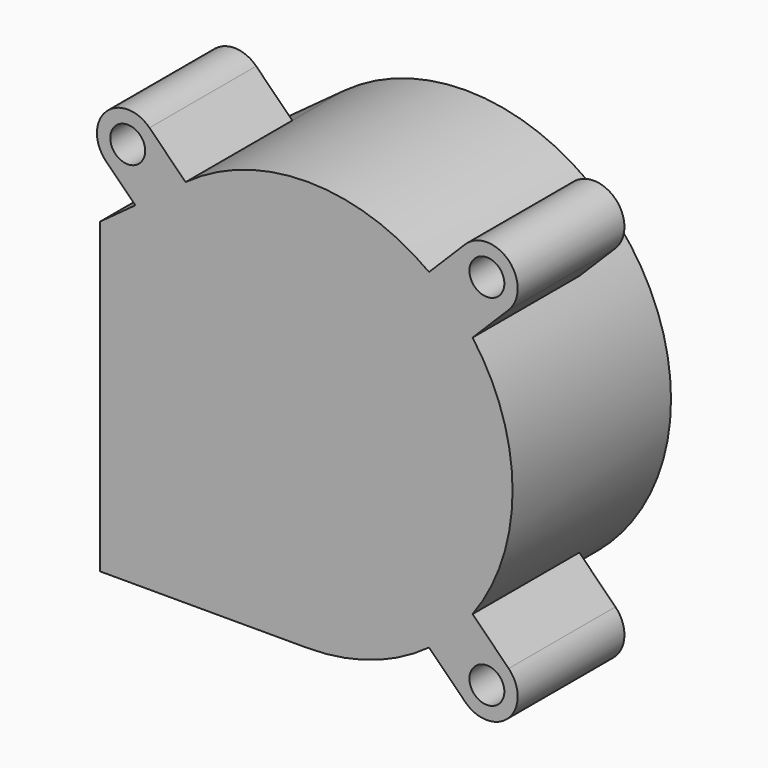
from build123d import *

# Parameters (mm, degrees)
F0_R     = 1.7
F1_DEPTH = 13
F2_DEPTH = 19.3
F3_R     = 13.5
F4_DEPTH = 5


# Not quite as in the source:
# - ends of sketch curves that miss each other by under 0.0002 mm in the source are joined


with BuildPart() as f1:
    # F0 (on Front) → F1 (new body)
    with BuildSketch(Plane.XZ):
        with BuildLine():
            Line((-20.2, -20), (0, -20))
            ThreePointArc((0, -20), (6.2422337367, -19.0009083461), (11.8608111105, -16.1034517977))
            ThreePointArc((11.8608111105, -16.1034517977), (14.1421356237, -14.1421356237), (16.1034517977, -11.8608111105))
            ThreePointArc((16.1034517977, -11.8608111105), (20, 0), (16.1034517977, 11.8608111105))
            ThreePointArc((16.1034517977, 11.8608111105), (14.1421356237, 14.1421356237), (11.8608111105, 16.1034517977))
            ThreePointArc((11.8608111105, 16.1034517977), (0.0300507716, 19.9999774238), (-11.8123654956, 16.1390216989))
            Line((-11.8123654956, 16.1390216989), (-11.8608644463, 16.1035246693))
            Line((-11.8608644463, 16.1035246693), (-16.7602440212, 12.517603334))
            Line((-16.7602440212, 12.517603334), (-20.2, 10))
            Line((-20.2, 10), (-20.2, -20))
        make_face()
        with BuildLine():
            ThreePointArc((16.1034517977, -11.8608111105), (14.1421356237, -14.1421356237), (11.8608111105, -16.1034517977))
            Line((11.8608111105, -16.1034517977), (15.3786796564, -19.6213203436))
            ThreePointArc((15.3786796564, -19.6213203436), (19.6213203436, -19.6213203436), (19.6213203436, -15.3786796564))
            Line((19.6213203436, -15.3786796564), (16.1034517977, -11.8608111105))
        make_face()
        with Locations((17.5, -17.5)):
            Circle(F0_R, mode=Mode.SUBTRACT)
        with BuildLine():
            ThreePointArc((11.8608111105, 16.1034517977), (14.1421356237, 14.1421356237), (16.1034517977, 11.8608111105))
            Line((16.1034517977, 11.8608111105), (19.6213203436, 15.3786796564))
            ThreePointArc((19.6213203436, 15.3786796564), (19.6213203436, 19.6213203436), (15.3786796564, 19.6213203436))
            Line((15.3786796564, 19.6213203436), (11.8608111105, 16.1034517977))
        make_face()
        with Locations((17.5, 17.5)):
            Circle(F0_R, mode=Mode.SUBTRACT)
        with BuildLine():
            Line((-19.6213203436, 15.3786796564), (-16.7602440212, 12.517603334))
            Line((-16.7602440212, 12.517603334), (-11.8608644463, 16.1035246693))
            Line((-11.8608644463, 16.1035246693), (-15.3786796564, 19.6213203436))
            ThreePointArc((-15.3786796564, 19.6213203436), (-19.6213203436, 19.6213203436), (-19.6213203436, 15.3786796564))
        make_face()
        with Locations((-17.5, 17.5)):
            Circle(F0_R, mode=Mode.SUBTRACT)
    extrude(amount=-F1_DEPTH)

    # F0 (on Front) → F2 (join)
    with BuildSketch(Plane.XZ):
        with BuildLine():
            Line((-20.2, -20), (0, -20))
            ThreePointArc((0, -20), (6.2422337367, -19.0009083461), (11.8608111105, -16.1034517977))
            ThreePointArc((11.8608111105, -16.1034517977), (14.1421356237, -14.1421356237), (16.1034517977, -11.8608111105))
            ThreePointArc((16.1034517977, -11.8608111105), (20, 0), (16.1034517977, 11.8608111105))
            ThreePointArc((16.1034517977, 11.8608111105), (14.1421356237, 14.1421356237), (11.8608111105, 16.1034517977))
            ThreePointArc((11.8608111105, 16.1034517977), (0.0300507716, 19.9999774238), (-11.8123654956, 16.1390216989))
            Line((-11.8123654956, 16.1390216989), (-11.8608644463, 16.1035246693))
            Line((-11.8608644463, 16.1035246693), (-16.7602440212, 12.517603334))
            Line((-16.7602440212, 12.517603334), (-20.2, 10))
            Line((-20.2, 10), (-20.2, -20))
        make_face()
    extrude(amount=-F2_DEPTH)

    # F3 (on face) → F4 (cut)
    with BuildSketch(Plane(origin=(0, 19.3, 0), x_dir=(-1, 0, 0), z_dir=(0, 1, 0))):
        with Locations((0, 1.5)):
            Circle(F3_R)
    extrude(amount=-F4_DEPTH, mode=Mode.SUBTRACT)


solid = f1.part
